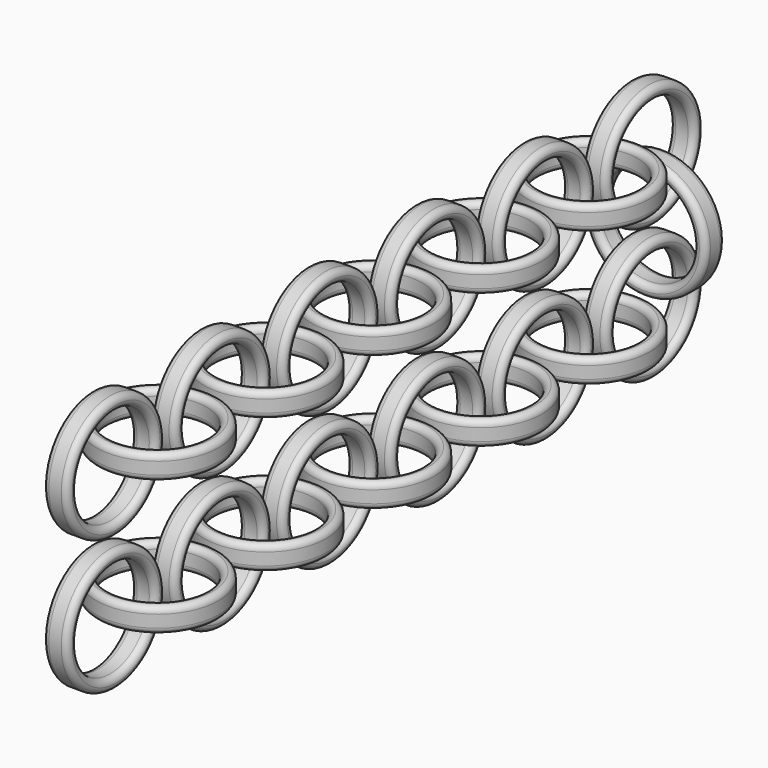
from build123d import *

# Parameters (mm, degrees)
F0_R      = 10
F0_R_2    = 8
F1_DEPTH  = 2
F2_R      = 0.99999
F3_R      = 0.99999
F10_R     = 10
F10_R_2   = 8
F11_DEPTH = 2
F12_R     = 0.99999
F29_R     = 10
F29_R_2   = 8
F30_DEPTH = 2
F31_R     = 0.99999


# Not quite as in the source:
# - a fillet or chamfer is up to 0.001 mm smaller than in the source, because OpenCascade refuses the exact size


with BuildPart() as f1:
    # F0 (on Top) → F1 (new body, symmetric)
    with BuildSketch(Plane.XY):
        Circle(F0_R)
        Circle(F0_R_2, mode=Mode.SUBTRACT)
    extrude(amount=F1_DEPTH, both=True)

    # F2 (radius 1 in the source; OpenCascade refuses exactly that, so slightly less here)
    f2_edges = [f1.edges().sort_by_distance(p)[0] for p in [
        (-10, 0, 2),
        (-8, 0, 2),
    ]]
    fillet(f2_edges, radius=F2_R)

    # F3 (radius 1 in the source; OpenCascade refuses exactly that, so slightly less here)
    f3_edges = [f1.edges().sort_by_distance(p)[0] for p in [
        (-10, 0, -2),
        (-8, 0, -2),
    ]]
    fillet(f3_edges, radius=F3_R)


with BuildPart() as f4_1:
    # F4: copy of F1
    add(f1.part.moved(Location((0, 22, 0))))


with BuildPart() as f5_1:
    # F5: copy of F1
    add(f1.part.moved(Location((0, 44, 0))))


with BuildPart() as f6_1:
    # F6: copy of F1
    add(f1.part.moved(Location((0, -22, 0))))


with BuildPart() as f7_1:
    # F7: copy of F1
    add(f1.part.moved(Location((0, -44, 0))))


with BuildPart() as f8_1:
    # F8: copy of F1
    add(f1.part.moved(Location((0, -10.6, 0.3))))


with BuildPart() as f11:
    # F10 (on Right) → F11 (new body, symmetric)
    with BuildSketch(Plane.YZ):
        with Locations((-10.9231067065, 0)):
            Circle(F10_R)
        with Locations((-10.9231067065, 0)):
            Circle(F10_R_2, mode=Mode.SUBTRACT)
    extrude(amount=F11_DEPTH, both=True)

    # F12 (radius 1 in the source; OpenCascade refuses exactly that, so slightly less here)
    f12_edges = [f11.edges().sort_by_distance(p)[0] for p in [
        (2, -20.923107, 0),
        (2, -18.923107, 0),
        (-2, -18.923107, 0),
        (-2, -20.923107, 0),
    ]]
    fillet(f12_edges, radius=F12_R)


with BuildPart() as f13_1:
    # F13: copy of F11
    add(f11.part.moved(Location((0, 22, 0))))


with BuildPart() as f14_1:
    # F14: copy of F11
    add(f11.part.moved(Location((0, 44, 0))))


with BuildPart() as f15_1:
    # F15: copy of F11
    add(f11.part.moved(Location((0, -22, 0))))


with BuildPart() as f16_1:
    # F16: copy of F11
    add(f11.part.moved(Location((0, -44, 0))))


with BuildPart() as f17_1:
    # F17: copy of F11
    add(f11.part.moved(Location((0, 66, 0))))


with BuildPart() as f18_1:
    # F18: copy of F16_1
    add(f16_1.part.moved(Location((0, 0, 22))))


with BuildPart() as f19_1:
    # F19: copy of F18_1
    add(f18_1.part.moved(Location((0, 22, 0))))


with BuildPart() as f20_1:
    # F20: copy of F19_1
    add(f19_1.part.moved(Location((0, 22, 0))))


with BuildPart() as f21_1:
    # F21: copy of F19_1
    add(f19_1.part.moved(Location((0, 44, 0))))


with BuildPart() as f22_1:
    # F22: copy of F20_1
    add(f20_1.part.moved(Location((0, 44, 0))))


with BuildPart() as f23_1:
    # F23: copy of F20_1
    add(f20_1.part.moved(Location((0, 66, 0))))


with BuildPart() as f24_1:
    # F24: copy of F7_1
    add(f7_1.part.moved(Location((0, 0, 22))))


with BuildPart() as f25_1:
    # F25: copy of F24_1
    add(f24_1.part.moved(Location((0, 22, 0))))


with BuildPart() as f26_1:
    # F26: copy of F24_1
    add(f24_1.part.moved(Location((0, 44, 0))))


with BuildPart() as f27_1:
    # F27: copy of F24_1
    add(f24_1.part.moved(Location((0, 66, 0))))


with BuildPart() as f28_1:
    # F28: copy of F24_1
    add(f24_1.part.moved(Location((0, 88, 0))))


with BuildPart() as f30:
    # F29 (on Front) → F30 (new body, symmetric)
    with BuildSketch(Plane.XZ):
        with Locations((0, 10.8798859734)):
            Circle(F29_R)
        with Locations((0, 10.8798859734)):
            Circle(F29_R_2, mode=Mode.SUBTRACT)
    extrude(amount=F30_DEPTH, both=True)

    # F31 (radius 1 in the source; OpenCascade refuses exactly that, so slightly less here)
    f31_edges = [f30.edges().sort_by_distance(p)[0] for p in [
        (-8, -2, 10.879886),
        (-10, -2, 10.879886),
        (-10, 2, 10.879886),
        (-8, 2, 10.879886),
    ]]
    fillet(f31_edges, radius=F31_R)


with BuildPart() as f32_1:
    # F32: copy of F30
    add(f30.part.moved(Location((0, 57.4, 0))))


solid = Compound([f1.part, f4_1.part, f5_1.part, f6_1.part, f7_1.part, f11.part, f13_1.part, f14_1.part, f15_1.part, f16_1.part, f17_1.part, f18_1.part, f19_1.part, f20_1.part, f21_1.part, f22_1.part, f23_1.part, f24_1.part, f25_1.part, f26_1.part, f27_1.part, f28_1.part, f32_1.part])
